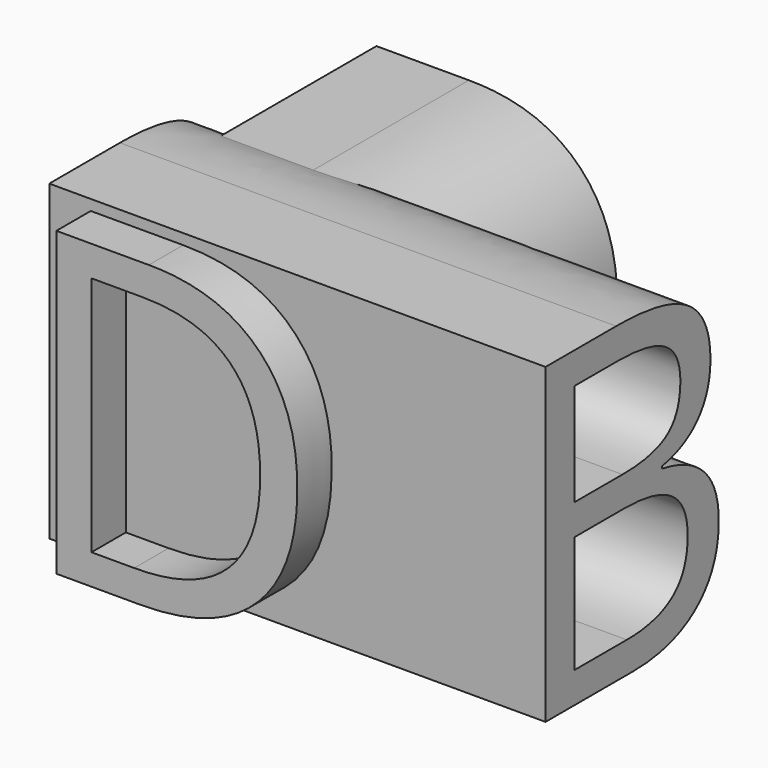
from build123d import *

# Parameters (mm, degrees)
F0_TEXT_SIZE = 104.7059479687
F2_DEPTH     = 99.0509614348
F1_TEXT_SIZE = 108.3881076839
F3_DEPTH     = 122.8793859482


# Not quite as in the source:
# - Text() gives the source's letters only with a copy of the font that has no kerning and outlines rounded to 1/6400 em; it was checked with that copy


with BuildPart() as f2:
    # F0 (on Front) → F2 (new body)
    with BuildSketch(Plane.XZ):
        with Locations((0, 0)):
            Text('D', F0_TEXT_SIZE, font='Open Sans', text_align=(TextAlign.LEFT, TextAlign.BOTTOM))
    extrude(amount=-F2_DEPTH)

    # F1 (on Right) → F3 (join)
    with BuildSketch(Plane.YZ):
        with Locations((0, 0)):
            Text('B', F1_TEXT_SIZE, font='Open Sans', text_align=(TextAlign.LEFT, TextAlign.BOTTOM))
    extrude(amount=F3_DEPTH)


solid = f2.part
